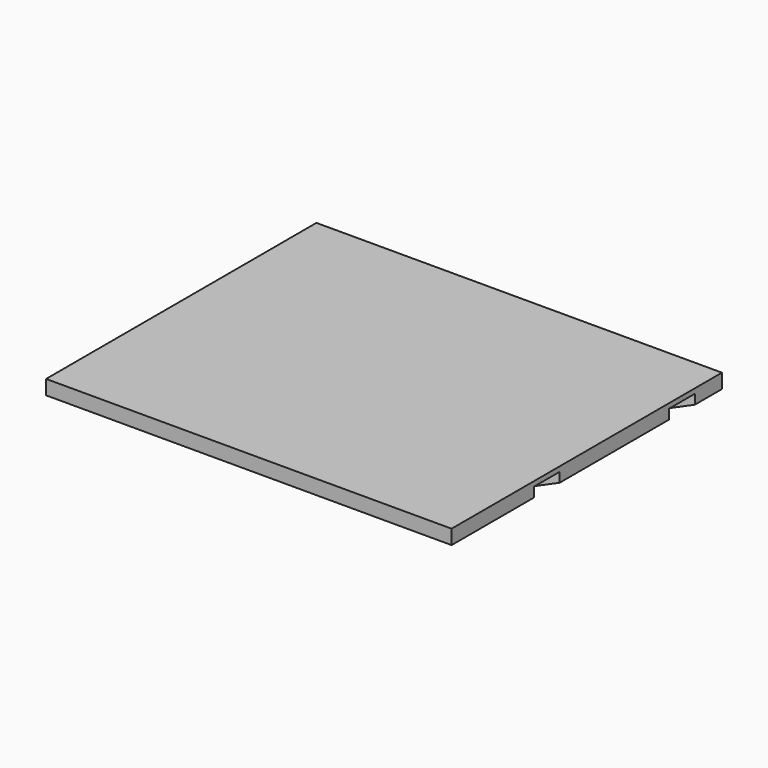
from build123d import *

# Parameters (mm, degrees)
F1_DEPTH = 70
F3_DEPTH = 2


# Not quite as in the source:
# - a feature names something its author has since deleted; it is built from what else it names


with BuildPart() as f1:
    # F0 (on Front) → F1 (new body)
    with BuildSketch(Plane.XZ):
        Polygon((0, -20), (0, -23), (32, -23), (32, -21), (38, -21), (42, -21), (42, -20), align=None)
        Polygon((-32, -23), (0, -23), (0, -20), (-17, -20), (-21, -20), (-30, -20), (-34, -20), (-34, -21), (-32, -21), align=None)
        Polygon((32, -21), (32, -23), (38, -23), (38, -22.25), (38, -21), align=None)
        Polygon((-38, -23), (-32, -23), (-32, -21), (-34, -21), (-38, -21), (-38, -22.25), align=None)
        Polygon((38, -22.25), (38, -23), (42, -23), (42, -21), (38, -21), align=None)
        Polygon((-42, -23), (-38, -23), (-38, -22.25), (-38, -21), (-42, -21), align=None)
        Polygon((-38, -21), (-34, -21), (-34, -20), (-42, -20), (-42, -21), align=None)
    extrude(amount=F1_DEPTH)

    # F2 (on face) → F3 (cut)
    with BuildSketch(Plane(origin=(0, 0, -23), x_dir=(1, 0, 0), z_dir=(0, 0, -1))):
        Polygon((42, 42), (42, 48.7185199326), (32, 63), (32, 56.2814800674), align=None)
        Polygon((42, 7), (42, 13.7185199326), (32, 28), (32, 21.2814800674), align=None)
    extrude(amount=-F3_DEPTH, mode=Mode.SUBTRACT)


solid = f1.part
